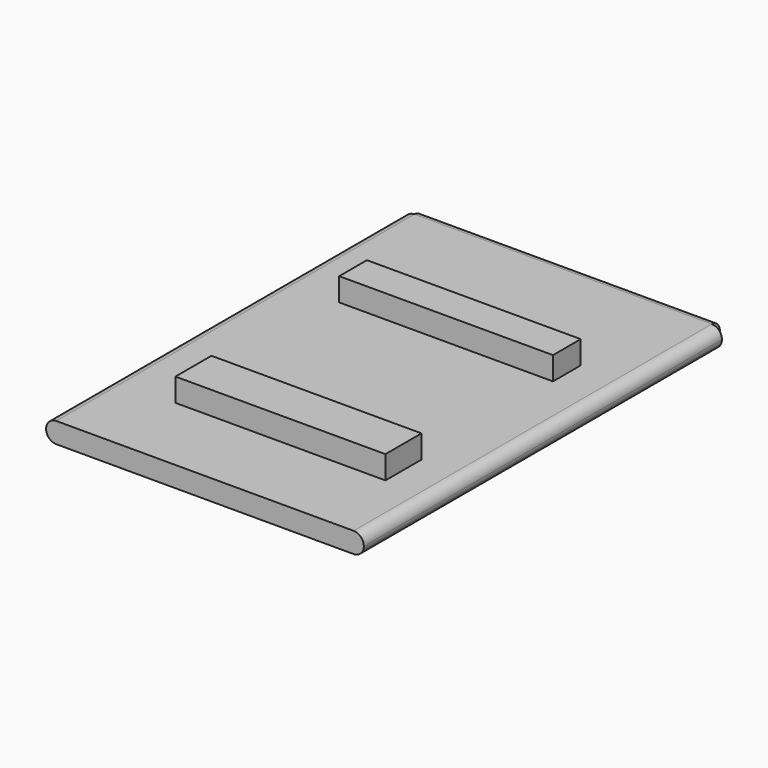
from build123d import *

# Parameters (mm, degrees)
F0_W     = 25.7
F0_H     = 38.7
F1_DEPTH = 1.77
F4_DEPTH = 38.7
F5_DEPTH = 25.7
F6_W     = 18.1557917967
F6_H     = 3.8920287043
F6_W_2   = 18.4808271006
F6_H_2   = 2.9954407364
F7_DEPTH = 2


with BuildPart() as f1:
    # F0 (on Top) → F1 (new body)
    with BuildSketch(Plane.XY):
        with Locations((12.85, -19.35)):
            Rectangle(F0_W, F0_H)
    extrude(amount=F1_DEPTH)

    # F2 (on face) → F4 (join)
    with BuildSketch(Plane.XZ.offset(38.7)):
        with BuildLine():
            ThreePointArc((25.7, 0), (26.3257895014, 0.2592104986), (26.585, 0.885))
            ThreePointArc((26.585, 0.885), (26.3257895014, 1.5107895014), (25.7, 1.77))
            Line((25.7, 1.77), (25.7, 0))
        make_face()
        with BuildLine():
            Line((25.7, 0), (25.7, 1.77))
            ThreePointArc((25.7, 1.77), (24.815, 0.885), (25.7, 0))
        make_face()
        with BuildLine():
            Line((0, 0), (0, 1.77))
            ThreePointArc((0, 1.77), (-0.885, 0.885), (0, 0))
        make_face()
    extrude(amount=-F4_DEPTH)

    # F3 (on face) → F5 (join)
    with BuildSketch(Plane.YZ.offset(25.7)):
        with BuildLine():
            ThreePointArc((0, 0), (0.6257895014, 0.2592104986), (0.885, 0.885))
            ThreePointArc((0.885, 0.885), (0.6257895014, 1.5107895014), (0, 1.77))
            Line((0, 1.77), (0, 0))
        make_face()
        with BuildLine():
            Line((0, 0), (0, 1.77))
            ThreePointArc((0, 1.77), (-0.885, 0.885), (0, 0))
        make_face()
    extrude(amount=-F5_DEPTH)

    # F6 (on face) → F7 (join)
    with BuildSketch(Plane.XY.offset(1.77)):
        with Locations((13.7009262107, -29.6595497057)):
            Rectangle(F6_W, F6_H)
        with Locations((13.3267915808, -11.7375161499)):
            Rectangle(F6_W_2, F6_H_2)
    extrude(amount=F7_DEPTH)


solid = f1.part
